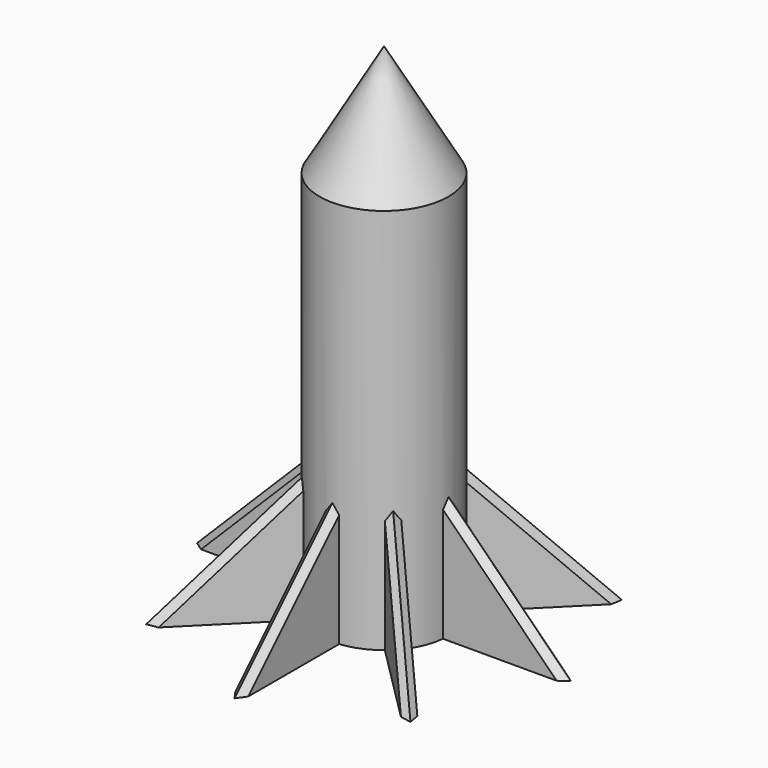
from build123d import *

# Parameters (mm, degrees)
F0_R      = 12.7
F1_DEPTH  = 76.2
F1_FACE_R = 12.7
F2_DEPTH  = 25.4
F2_TAPER  = 30
F3_T      = -2.54
F5_DEPTH  = 1.27
F6_SIZE   = 1.2699
F7_COUNT  = 8


# Not quite as in the source:
# - a fillet or chamfer is up to 0.001 mm smaller than in the source, because OpenCascade refuses the exact size


with BuildPart() as f1:
    # F0 (on Top) → F1 (new body)
    with BuildSketch(Plane.XY):
        Circle(F0_R)
    extrude(amount=F1_DEPTH)

    # F1_face (on face) → F2 (join)
    with BuildSketch(Plane.XY.offset(76.2)):
        Circle(F1_FACE_R)
    extrude(amount=F2_DEPTH, taper=F2_TAPER)

    # F3
    f3_openings = [f1.faces().sort_by_distance(p)[0] for p in [
        (0, 0, 0),
    ]]
    offset(amount=F3_T, openings=f3_openings)

    # F4 (on Front) → F5 (join, symmetric)
    with BuildSketch(Plane.XZ):
        Polygon((-11.43, 25.4), (-36.83, 0), (-11.43, 0), align=None)
    extrude(amount=F5_DEPTH, both=True)

    # F6 (size 1.27 in the source; OpenCascade refuses exactly that, so slightly less here)
    f6_edges = [f1.edges().sort_by_distance(p)[0] for p in [
        (-24.73317, -1.27, 12.09683),
        (-24.73317, 1.27, 12.09683),
    ]]
    chamfer(f6_edges, length=F6_SIZE)

    # F7: F1 ×8 about axis
    f7_axis = Axis((0, 0, 0), (0, 0, 1))


with BuildPart() as f1_1:
    add(f1.part)
    for i in range(1, F7_COUNT):
        add(f1.part.rotate(f7_axis, i * 360 / F7_COUNT))


solid = f1_1.part
